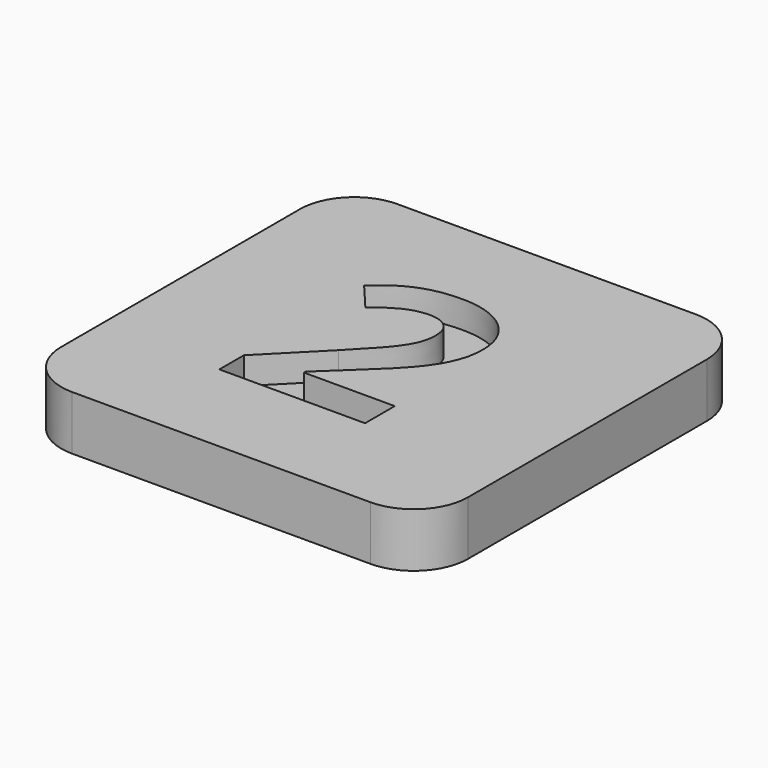
from build123d import *

# Parameters (mm, degrees)
F0_W         = 38.1
F0_H         = 38.1
F1_DEPTH     = 5.08
F2_TEXT_SIZE = 27.3386804657
F3_DEPTH     = 2.54
F4_R         = 5.08


# Not quite as in the source:
# - Text() gives the source's letters only with a copy of the font that has no kerning and outlines rounded to 1/6400 em; it was checked with that copy


with BuildPart() as f1:
    # F0 (on Top) → F1 (new body)
    with BuildSketch(Plane.XY):
        Rectangle(F0_W, F0_H)
    extrude(amount=F1_DEPTH)

    # F2 (on face) → F3 (cut)
    with BuildSketch(Plane.XY.offset(5.08)):
        with Locations((-8.89, -9.525)):
            Text('2', F2_TEXT_SIZE, font='Open Sans', font_style=FontStyle.BOLD, text_align=(TextAlign.LEFT, TextAlign.BOTTOM))
    extrude(amount=-F3_DEPTH, mode=Mode.SUBTRACT)

    # F4
    f4_edges = [f1.edges().sort_by_distance(p)[0] for p in [
        (-19.05, -19.05, 2.54),
        (19.05, -19.05, 2.54),
        (19.05, 19.05, 2.54),
        (-19.05, 19.05, 2.54),
    ]]
    fillet(f4_edges, radius=F4_R)


solid = f1.part
